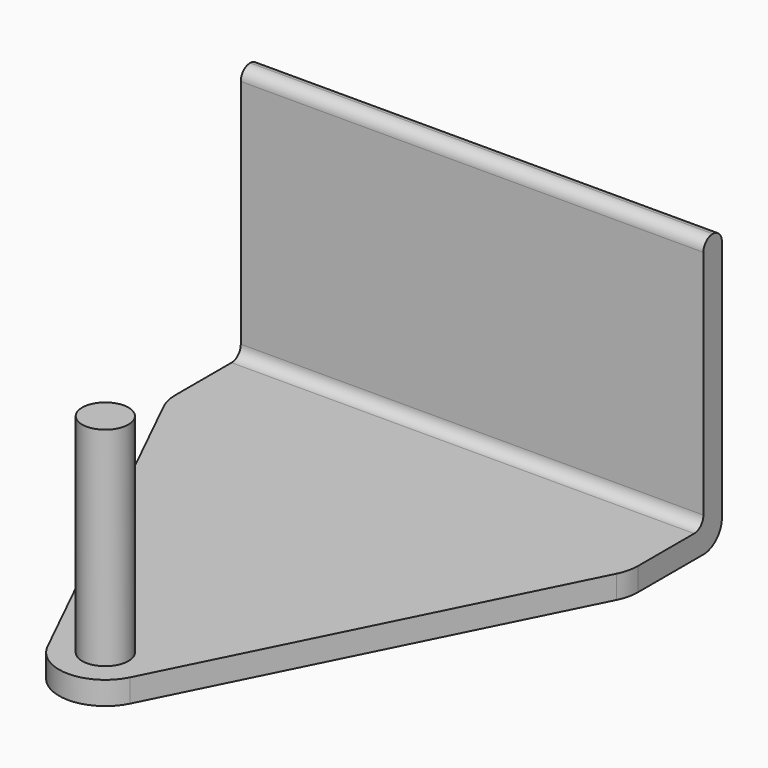
from build123d import *

# Parameters (mm, degrees)
F0_W     = 200
F0_H     = 50
F1_DEPTH = 10
F2_R     = 20
F3_R     = 10
F4_DEPTH = 90
F5_W     = 200
F5_H     = 10
F6_DEPTH = 110
F7_R     = 4.99999
F8_R     = 10


# Not quite as in the source:
# - a fillet or chamfer is up to 0.001 mm smaller than in the source, because OpenCascade refuses the exact size


with BuildPart() as f1:
    # F0 (on Top) → F1 (new body)
    with BuildSketch(Plane.XY):
        Polygon((200, 0), (0, 0), (98.8994031925, -202.201193615), align=None)
        with Locations((100, 25)):
            Rectangle(F0_W, F0_H)
    extrude(amount=F1_DEPTH)

    # F2
    f2_edges = [f1.edges().sort_by_distance(p)[0] for p in [
        (98.899403, -202.201194, 5),
        (200, 0, 5),
        (0, 0, 5),
    ]]
    fillet(f2_edges, radius=F2_R)

    # F3 (on face) → F4 (join)
    with BuildSketch(Plane.XY.offset(10)):
        with Locations((99.0967144561, -157.0852115379)):
            Circle(F3_R)
    extrude(amount=F4_DEPTH)

    # F5 (on face) → F6 (join)
    with BuildSketch(Plane.XY.offset(10)):
        with Locations((100, 45)):
            Rectangle(F5_W, F5_H)
    extrude(amount=F6_DEPTH)

    # F7 (radius 5 in the source; OpenCascade refuses exactly that, so slightly less here)
    f7_edges = [f1.edges().sort_by_distance(p)[0] for p in [
        (100, 50, 120),
        (100, 40, 120),
        (100, 40, 10),
    ]]
    fillet(f7_edges, radius=F7_R)

    # F8
    f8_edges = [f1.edges().sort_by_distance(p)[0] for p in [
        (100, 50, 0),
    ]]
    fillet(f8_edges, radius=F8_R)


solid = f1.part
